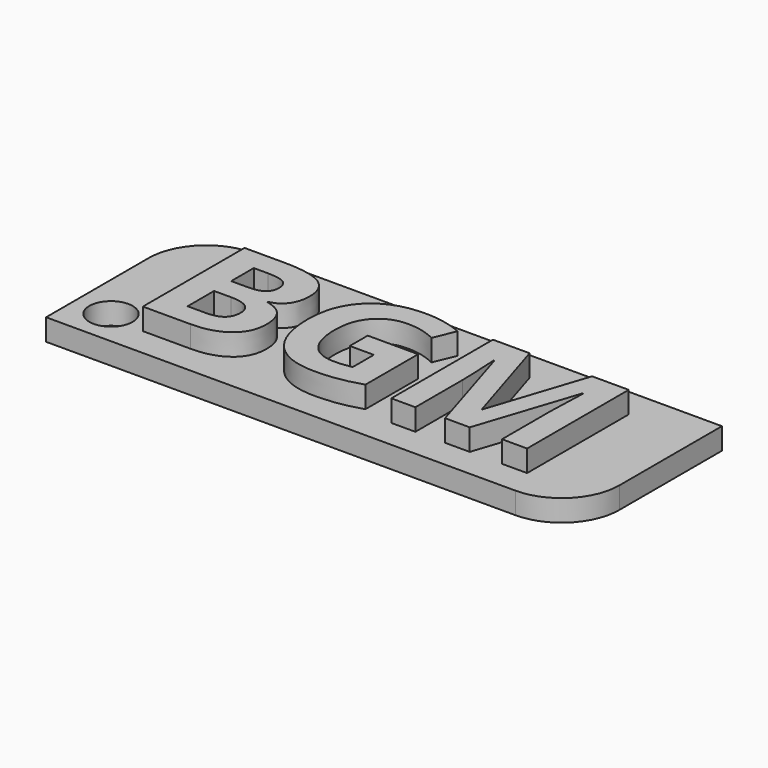
from build123d import *

# Parameters (mm, degrees)
F0_TEXT_SIZE = 12.3355272485
F1_DEPTH     = 3
F0_R         = 1.5
F2_DEPTH     = 1.5


# Not quite as in the source:
# - Text() gives the source's letters only with a copy of the font that has no kerning and outlines rounded to 1/6400 em; it was checked with that copy


with BuildPart() as f1:
    # F0 (on Top) → F1 (new body)
    with BuildSketch(Plane.XY):
        with Locations((4, 2)):
            Text('BGM', F0_TEXT_SIZE, font='Open Sans', font_style=FontStyle.BOLD, text_align=(TextAlign.LEFT, TextAlign.BOTTOM))
    extrude(amount=F1_DEPTH)

    # F0 (on Top) → F2 (join)
    with BuildSketch(Plane.XY):
        with BuildLine():
            Line((0, 8.8815796189), (0, 0))
            Line((0, 0), (32.5413261712, 0))
            ThreePointArc((32.5413261712, 0), (35.3697532959, 1.1715728753), (36.5413261712, 4))
            Line((36.5413261712, 4), (36.5413261712, 12.8815796189))
            Line((36.5413261712, 12.8815796189), (4, 12.8815796189))
            ThreePointArc((4, 12.8815796189), (1.1715728753, 11.7100067436), (0, 8.8815796189))
        make_face()
        with Locations((2.5, 2.5)):
            Circle(F0_R, mode=Mode.SUBTRACT)
        with BuildLine():
            Line((5.1082700262, 2), (5.1082700262, 10.8064099997))
            Line((5.1082700262, 10.8064099997), (7.8490699868, 10.8064099997))
            add(Edge.make_bspline(
                [(7.8490699868, 10.8064099997), (9.7225281876, 10.8064099997), (10.5686682598, 10.2734766741)],
                knots=[0, 0, 0, 1, 1, 1], degree=2))
            add(Edge.make_bspline(
                [(10.5686682598, 10.2734766741), (11.414808332, 9.7405433484), (11.414808332, 8.5783053905)],
                knots=[0, 0, 0, 1, 1, 1], degree=2))
            add(Edge.make_bspline(
                [(11.414808332, 8.5783053905), (11.414808332, 7.7880606761), (11.0447425146, 7.2821113163)],
                knots=[0, 0, 0, 1, 1, 1], degree=2))
            add(Edge.make_bspline(
                [(11.0447425146, 7.2821113163), (10.6746766971, 6.7761619565), (10.0598277608, 6.6740083715)],
                knots=[0, 0, 0, 1, 1, 1], degree=2))
            Line((10.0598277608, 6.6740083715), (10.0598277608, 6.6142581614))
            add(Edge.make_bspline(
                [(10.0598277608, 6.6142581614), (10.8963307023, 6.4272978265), (11.2673602329, 5.9155661883)],
                knots=[0, 0, 0, 1, 1, 1], degree=2))
            add(Edge.make_bspline(
                [(11.2673602329, 5.9155661883), (11.6383897634, 5.4038345501), (11.6383897634, 4.5538396257)],
                knots=[0, 0, 0, 1, 1, 1], degree=2))
            add(Edge.make_bspline(
                [(11.6383897634, 4.5538396257), (11.6383897634, 3.3491982928), (10.7671931515, 2.6745991464)],
                knots=[0, 0, 0, 1, 1, 1], degree=2))
            add(Edge.make_bspline(
                [(10.7671931515, 2.6745991464), (9.8959965395, 2), (8.4022412868, 2)],
                knots=[0, 0, 0, 1, 1, 1], degree=2))
            Line((8.4022412868, 2), (5.1082700262, 2))
        make_face(mode=Mode.SUBTRACT)
        with BuildLine():
            Line((16.7383593102, 5.3903425672), (16.7383593102, 6.9457754562))
            Line((16.7383593102, 6.9457754562), (20.2327828885, 6.9457754562))
            Line((20.2327828885, 6.9457754562), (20.2327828885, 2.3797029481))
            add(Edge.make_bspline(
                [(20.2327828885, 2.3797029481), (19.3827879641, 2.102153585), (18.6330191985, 1.9903628693)],
                knots=[0, 0, 0, 1, 1, 1], degree=2))
            add(Edge.make_bspline(
                [(18.6330191985, 1.9903628693), (17.8832504329, 1.8785721536), (17.1007154231, 1.8785721536)],
                knots=[0, 0, 0, 1, 1, 1], degree=2))
            add(Edge.make_bspline(
                [(17.1007154231, 1.8785721536), (15.107756802, 1.8785721536), (14.0563458467, 3.0504472423)],
                knots=[0, 0, 0, 1, 1, 1], degree=2))
            add(Edge.make_bspline(
                [(14.0563458467, 3.0504472423), (13.0049348914, 4.2223223309), (13.0049348914, 6.4157332697)],
                knots=[0, 0, 0, 1, 1, 1], degree=2))
            add(Edge.make_bspline(
                [(13.0049348914, 6.4157332697), (13.0049348914, 8.5474665724), (14.2249956333, 9.7395796354)],
                knots=[0, 0, 0, 1, 1, 1], degree=2))
            add(Edge.make_bspline(
                [(14.2249956333, 9.7395796354), (15.4450563752, 10.9316926983), (17.6057010698, 10.9316926983)],
                knots=[0, 0, 0, 1, 1, 1], degree=2))
            add(Edge.make_bspline(
                [(17.6057010698, 10.9316926983), (18.9626090672, 10.9316926983), (20.2212183317, 10.3900859551)],
                knots=[0, 0, 0, 1, 1, 1], degree=2))
            Line((20.2212183317, 10.3900859551), (19.6005871171, 8.8963307023))
            add(Edge.make_bspline(
                [(19.6005871171, 8.8963307023), (18.6368740508, 9.3781872355), (17.594136513, 9.3781872355)],
                knots=[0, 0, 0, 1, 1, 1], degree=2))
            add(Edge.make_bspline(
                [(17.594136513, 9.3781872355), (16.3837129018, 9.3781872355), (15.6551458237, 8.5648134075)],
                knots=[0, 0, 0, 1, 1, 1], degree=2))
            add(Edge.make_bspline(
                [(15.6551458237, 8.5648134075), (14.9265787456, 7.7514395796), (14.9265787456, 6.3791121732)],
                knots=[0, 0, 0, 1, 1, 1], degree=2))
            add(Edge.make_bspline(
                [(14.9265787456, 6.3791121732), (14.9265787456, 4.9451071306), (15.5134800029, 4.1895560866)],
                knots=[0, 0, 0, 1, 1, 1], degree=2))
            add(Edge.make_bspline(
                [(15.5134800029, 4.1895560866), (16.1003812603, 3.4340050426), (17.2202158433, 3.4340050426)],
                knots=[0, 0, 0, 1, 1, 1], degree=2))
            add(Edge.make_bspline(
                [(17.2202158433, 3.4340050426), (17.8061533876, 3.4340050426), (18.407510341, 3.5535054629)],
                knots=[0, 0, 0, 1, 1, 1], degree=2))
            Line((18.407510341, 3.5535054629), (18.407510341, 5.3903425672))
            Line((18.407510341, 5.3903425672), (16.7383593102, 5.3903425672))
        make_face(mode=Mode.SUBTRACT)
        with BuildLine():
            Line((27.7670916408, 2), (26.055537235, 2))
            Line((26.055537235, 2), (23.9353684892, 8.9078952591))
            Line((23.9353684892, 8.9078952591), (23.8814005575, 8.9078952591))
            add(Edge.make_bspline(
                [(23.8814005575, 8.9078952591), (23.9970461255, 6.8012184962), (23.9970461255, 6.0957805317)],
                knots=[0, 0, 0, 1, 1, 1], degree=2))
            Line((23.9970461255, 6.0957805317), (23.9970461255, 2))
            Line((23.9970461255, 2), (22.3278950946, 2))
            Line((22.3278950946, 2), (22.3278950946, 10.8064099997))
            Line((22.3278950946, 10.8064099997), (24.8701701635, 10.8064099997))
            Line((24.8701701635, 10.8064099997), (26.9537178128, 4.0719830925))
            Line((26.9537178128, 4.0719830925), (26.9903389093, 4.0719830925))
            Line((26.9903389093, 4.0719830925), (29.2010966834, 10.8064099997))
            Line((29.2010966834, 10.8064099997), (31.7414443261, 10.8064099997))
            Line((31.7414443261, 10.8064099997), (31.7414443261, 2))
            Line((31.7414443261, 2), (30.0009785284, 2))
            Line((30.0009785284, 2), (30.0009785284, 6.1690227248))
            add(Edge.make_bspline(
                [(30.0009785284, 6.1690227248), (30.0009785284, 6.463918923), (30.0106156591, 6.8494041496)],
                knots=[0, 0, 0, 1, 1, 1], degree=2))
            add(Edge.make_bspline(
                [(30.0106156591, 6.8494041496), (30.0202527897, 7.2348893761), (30.0915675567, 8.8963307023)],
                knots=[0, 0, 0, 1, 1, 1], degree=2))
            Line((30.0915675567, 8.8963307023), (30.0375996249, 8.8963307023))
            Line((30.0375996249, 8.8963307023), (27.7670916408, 2))
        make_face(mode=Mode.SUBTRACT)
        with BuildLine():
            Line((8.1324016282, 5.83750543), (6.9759459487, 5.83750543))
            Line((6.9759459487, 5.83750543), (6.9759459487, 3.5419409061))
            Line((6.9759459487, 3.5419409061), (8.1921518383, 3.5419409061))
            add(Edge.make_bspline(
                [(8.1921518383, 3.5419409061), (8.9631222914, 3.5419409061), (9.3302969696, 3.8368371043)],
                knots=[0, 0, 0, 1, 1, 1], degree=2))
            add(Edge.make_bspline(
                [(9.3302969696, 3.8368371043), (9.6974716479, 4.1317333026), (9.6974716479, 4.7407999605)],
                knots=[0, 0, 0, 1, 1, 1], degree=2))
            add(Edge.make_bspline(
                [(9.6974716479, 4.7407999605), (9.6974716479, 5.83750543), (8.1324016282, 5.83750543)],
                knots=[0, 0, 0, 1, 1, 1], degree=2))
        make_face()
        with BuildLine():
            Line((6.9759459487, 9.2760336505), (6.9759459487, 7.3177686998))
            Line((6.9759459487, 7.3177686998), (8.0591594352, 7.3177686998))
            add(Edge.make_bspline(
                [(8.0591594352, 7.3177686998), (8.8185653314, 7.3177686998), (9.1587560438, 7.5529146879)],
                knots=[0, 0, 0, 1, 1, 1], degree=2))
            add(Edge.make_bspline(
                [(9.1587560438, 7.5529146879), (9.4989467562, 7.7880606761), (9.4989467562, 8.3296674194)],
                knots=[0, 0, 0, 1, 1, 1], degree=2))
            add(Edge.make_bspline(
                [(9.4989467562, 8.3296674194), (9.4989467562, 8.8365804922), (9.1288809388, 9.0563070714)],
                knots=[0, 0, 0, 1, 1, 1], degree=2))
            add(Edge.make_bspline(
                [(9.1288809388, 9.0563070714), (8.7588151213, 9.2760336505), (7.9570058502, 9.2760336505)],
                knots=[0, 0, 0, 1, 1, 1], degree=2))
            Line((7.9570058502, 9.2760336505), (6.9759459487, 9.2760336505))
        make_face()
    extrude(amount=F2_DEPTH)


solid = f1.part
